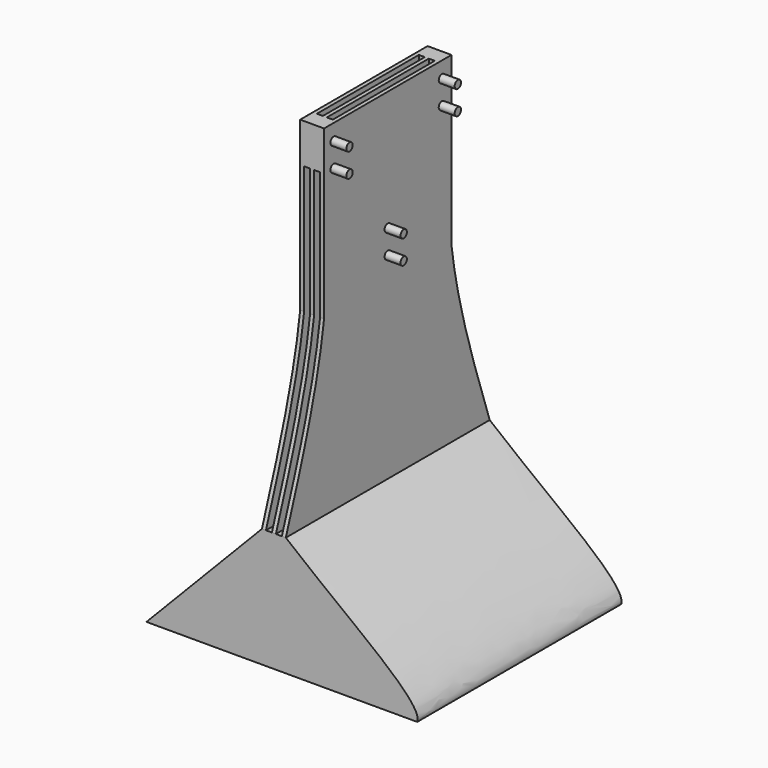
from build123d import *

# Parameters (mm, degrees)
F1_DEPTH  = 320
F2_W      = 30
F2_H      = 320
F3_DEPTH  = 428
F5_DEPTH  = 205
F7_W      = 260
F7_H      = 128.6325914682
F8_DEPTH  = 30
F9_W      = 7.5
F9_H      = 457.219858036
F10_DEPTH = 977
F6_W      = 20
F6_H      = 50
F6_H_2    = 25
F11_DEPTH = 25
F12_R     = 5.1978686685
F13_DEPTH = 63
F14_R     = 5
F15_DEPTH = 20


with BuildPart() as f1:
    # F0 (on Front) → F1 (new body)
    with BuildSketch(Plane.XZ):
        with BuildLine():
            Line((150.299176857, 1.1440683747), (180.299176857, 1.1440683747))
            Line((180.299176857, 1.1440683747), (340.299176857, 1.1440683747))
            add(Edge.make_bspline(
                [(340.299176857, 1.1440683747), (349.1569172885, 24.1151609846), (251.1032390966, 88.0444564268), (175.3079980464, 151.1440683747)],
                knots=[0.4586039165, 0.4586039165, 0.4586039165, 0.4586039165, 1, 1, 1, 1], degree=3))
            Line((175.3079980464, 151.1440683747), (145.3079980464, 151.1440683747))
            Line((145.3079980464, 151.1440683747), (0.299176857, 1.1440683747))
            Line((0.299176857, 1.1440683747), (100.299176857, 1.1440683747))
            Line((100.299176857, 1.1440683747), (150.299176857, 1.1440683747))
        make_face()
    extrude(amount=F1_DEPTH)

    # F2 (on face) → F3 (join)
    with BuildSketch(Plane.XY.offset(151.1440683747)):
        with Locations((160.3079980464, -160)):
            Rectangle(F2_W, F2_H)
    extrude(amount=F3_DEPTH)

    # F4 (on face) → F5 (cut)
    with BuildSketch(Plane(origin=(145.3079980464, 0, 0), x_dir=(0, -1, 0), z_dir=(-1, 0, 0))):
        with BuildLine():
            Line((0, 579.1440683747), (0, 151.1440683747))
            add(Edge.make_bspline(
                [(60, 368.6685562134), (50.1739969339, 296.0916949665), (25.086998467, 223.6178816706), (0, 151.1440683747)],
                knots=[0.4913001533, 0.4913001533, 0.4913001533, 0.4913001533, 1, 1, 1, 1], degree=3))
            Line((60, 368.6685562134), (60, 579.1440683747))
            Line((60, 579.1440683747), (0, 579.1440683747))
        make_face()
        with BuildLine():
            add(Edge.make_bspline(
                [(320, 151.1440683747), (294.913001533, 223.6178816706), (269.8260030661, 296.0916949665), (260, 368.6685562134)],
                knots=[0, 0, 0, 0, 0.5086998467, 0.5086998467, 0.5086998467, 0.5086998467], degree=3))
            Line((320, 151.1440683747), (320, 579.1440683747))
            Line((320, 579.1440683747), (260, 579.1440683747))
            Line((260, 579.1440683747), (260, 368.6685562134))
        make_face()
    extrude(amount=-F5_DEPTH, mode=Mode.SUBTRACT)

    # F7 (on face) → F8 (cut)
    with BuildSketch(Plane(origin=(-0.4170581217, 0, 0.4031807106), x_dir=(0, -1, 0), z_dir=(-0.7189672474, 0, 0.6950439534))):
        with Locations((160, 105.3467844897)):
            Rectangle(F7_W, F7_H)
    extrude(amount=-F8_DEPTH, mode=Mode.SUBTRACT)

    # F9 (on face) → F10 (cut)
    with BuildSketch(Plane.XZ.offset(320)):
        with Locations((154.0579980464, 379.7539973927)):
            Rectangle(F9_W, F9_H)
        with Locations((166.5579980464, 379.7539973927)):
            Rectangle(F9_W, F9_H)
    extrude(amount=-F10_DEPTH, mode=Mode.SUBTRACT)

    # F6 (on face) → F11 (join)
    with BuildSketch(Plane.YZ.offset(175.3079980464)):
        with Locations((-250, 554.1440683747)):
            Rectangle(F6_W, F6_H)
        with Locations((-70, 554.1440683747)):
            Rectangle(F6_W, F6_H)
        with Locations((-230, 406.1685562134)):
            Rectangle(F6_W, F6_H_2)
        with Locations((-90, 406.1685562134)):
            Rectangle(F6_W, F6_H_2)
    extrude(amount=-F11_DEPTH)

    # F12 (on Right) → F13 (cut)
    with BuildSketch(Plane.YZ):
        with Locations((-268.3978974819, 7.7915792353)):
            Circle(F12_R)
    extrude(amount=F13_DEPTH, mode=Mode.SUBTRACT)

    # F14 (on face) → F15 (join)
    with BuildSketch(Plane.YZ.offset(175.3079980464)):
        with Locations((-245, 559.1440683747)):
            Circle(F14_R)
        with Locations((-245, 529.1440683747)):
            Circle(F14_R)
        with Locations((-75, 559.1440683747)):
            Circle(F14_R)
        with Locations((-75, 529.1440683747)):
            Circle(F14_R)
        with Locations((-160, 428.5443711281)):
            Circle(F14_R)
        with Locations((-160, 398.5443711281)):
            Circle(F14_R)
    extrude(amount=F15_DEPTH)


solid = f1.part
